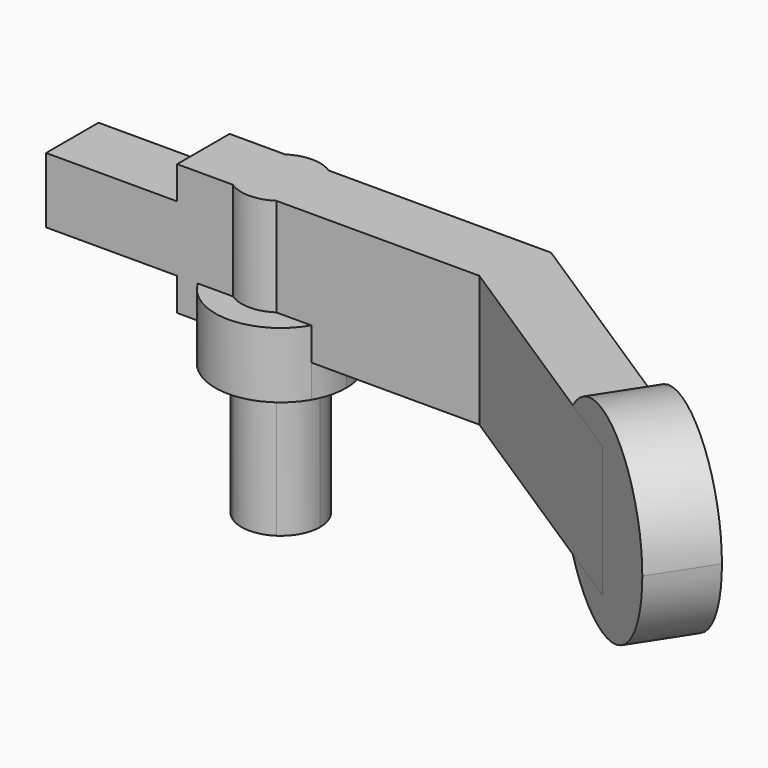
from build123d import *

# Parameters (mm, degrees)
F1_DEPTH = 12.7
F3_DEPTH = 15.875
F4_DEPTH = 3.175
F6_DEPTH = 6.349999961
F7_W     = 12.7
F7_H     = 3.175
F8_DEPTH = 9.526


with BuildPart() as f1:
    # F0 (on Top) → F1 (new body)
    with BuildSketch(Plane.XY):
        with BuildLine():
            ThreePointArc((2.1060567419, -3.175), (3.3570951868, -1.8016692001), (3.81, 0))
            ThreePointArc((3.81, 0), (3.3570951868, 1.8016692001), (2.1060567419, 3.175))
            ThreePointArc((2.1060567419, 3.175), (0, 3.81), (-2.1060567419, 3.175))
            ThreePointArc((-2.1060567419, 3.175), (-3.81, 0), (-2.1060567419, -3.175))
            ThreePointArc((-2.1060567419, -3.175), (0, -3.81), (2.1060567419, -3.175))
        make_face()
        with BuildLine():
            ThreePointArc((2.1060567419, 3.175), (3.3570951868, 1.8016692001), (3.81, 0))
            ThreePointArc((3.81, 0), (3.3570951868, -1.8016692001), (2.1060567419, -3.175))
            Line((2.1060567419, -3.175), (21.7762735865, -3.175))
            Line((21.7762735865, -3.175), (46.5216673911, -19.1860459745))
            Line((46.5216673911, -19.1860459745), (49.9712098046, -13.8547087462))
            Line((49.9712098046, -13.8547087462), (23.6514521839, 3.175))
            Line((23.6514521839, 3.175), (2.1060567419, 3.175))
        make_face()
        with BuildLine():
            ThreePointArc((-2.1060567419, -3.175), (-3.81, 0), (-2.1060567419, 3.175))
            Line((-2.1060567419, 3.175), (-20.2012713999, 3.175))
            Line((-20.2012713999, 3.175), (-20.2012713999, -3.175))
            Line((-20.2012713999, -3.175), (-2.1060567419, -3.175))
        make_face()
    extrude(amount=F1_DEPTH)

    # F2 (on face) → F3 (join)
    with BuildSketch(Plane(origin=(0, 0, 0), x_dir=(1, 0, 0), z_dir=(0, 0, -1))):
        with BuildLine():
            ThreePointArc((2.1060567419, -3.175), (3.3570951868, -1.8016692001), (3.81, 0))
            ThreePointArc((3.81, 0), (3.3570951868, 1.8016692001), (2.1060567419, 3.175))
            ThreePointArc((2.1060567419, 3.175), (0, 3.81), (-2.1060567419, 3.175))
            ThreePointArc((-2.1060567419, 3.175), (-3.81, 0), (-2.1060567419, -3.175))
            ThreePointArc((-2.1060567419, -3.175), (0, -3.81), (2.1060567419, -3.175))
        make_face()
    extrude(amount=F3_DEPTH)

    # F2 (on face) → F4 (join, symmetric)
    with BuildSketch(Plane(origin=(0, 0, 0), x_dir=(1, 0, 0), z_dir=(0, 0, -1))):
        with BuildLine():
            ThreePointArc((2.1060567419, 3.175), (3.3570951868, 1.8016692001), (3.81, 0))
            ThreePointArc((3.81, 0), (3.3570951868, -1.8016692001), (2.1060567419, -3.175))
            Line((2.1060567419, -3.175), (5.499261314, -3.175))
            ThreePointArc((5.499261314, -3.175), (6.1336289969, -1.6435009364), (6.35, 0))
            ThreePointArc((6.35, 0), (6.1336289969, 1.6435009364), (5.499261314, 3.175))
            Line((5.499261314, 3.175), (2.1060567419, 3.175))
        make_face()
        with BuildLine():
            ThreePointArc((-2.1060567419, 3.175), (0, 3.81), (2.1060567419, 3.175))
            Line((2.1060567419, 3.175), (5.499261314, 3.175))
            ThreePointArc((5.499261314, 3.175), (0, 6.35), (-5.499261314, 3.175))
            Line((-5.499261314, 3.175), (-2.1060567419, 3.175))
        make_face()
        with BuildLine():
            Line((5.499261314, -3.175), (2.1060567419, -3.175))
            ThreePointArc((2.1060567419, -3.175), (0, -3.81), (-2.1060567419, -3.175))
            Line((-2.1060567419, -3.175), (-5.499261314, -3.175))
            ThreePointArc((-5.499261314, -3.175), (0, -6.35), (5.499261314, -3.175))
        make_face()
        with BuildLine():
            ThreePointArc((-2.1060567419, -3.175), (-3.81, 0), (-2.1060567419, 3.175))
            Line((-2.1060567419, 3.175), (-5.499261314, 3.175))
            ThreePointArc((-5.499261314, 3.175), (-6.35, 0), (-5.499261314, -3.175))
            Line((-5.499261314, -3.175), (-2.1060567419, -3.175))
        make_face()
    extrude(amount=F4_DEPTH, both=True)

    # F5 (on face) → F6 (join, through all)
    with BuildSketch(Plane(origin=(4.9781873283, 7.6938887107, 0), x_dir=(0.839580671, -0.5432350291, 0), z_dir=(-0.5432350291, -0.839580671, 0))):
        with BuildLine():
            ThreePointArc((42.3817091402, 0), (52.8799553739, -2.5479917191), (59.0062249688, 6.35))
            ThreePointArc((59.0062249688, 6.35), (52.8799553739, 15.2479917191), (42.3817091402, 12.7))
            Line((42.3817091402, 12.7), (49.4812249688, 12.7))
            Line((49.4812249688, 12.7), (49.4812249688, 0))
            Line((49.4812249688, 0), (42.3817091402, 0))
        make_face()
        with BuildLine():
            Line((49.4812249688, 12.7), (42.3817091402, 12.7))
            ThreePointArc((42.3817091402, 12.7), (39.9562249688, 6.35), (42.3817091402, 0))
            Line((42.3817091402, 0), (49.4812249688, 0))
            Line((49.4812249688, 0), (49.4812249688, 12.7))
        make_face()
    extrude(amount=-F6_DEPTH)

    # F7 (on face) → F8 (cut, through all)
    with BuildSketch(Plane.XZ.offset(3.175)):
        with Locations((-13.8512713999, 11.1125)):
            Rectangle(F7_W, F7_H)
        with Locations((-13.8512713999, 1.5875)):
            Rectangle(F7_W, F7_H)
    extrude(amount=-F8_DEPTH, mode=Mode.SUBTRACT)


solid = f1.part
